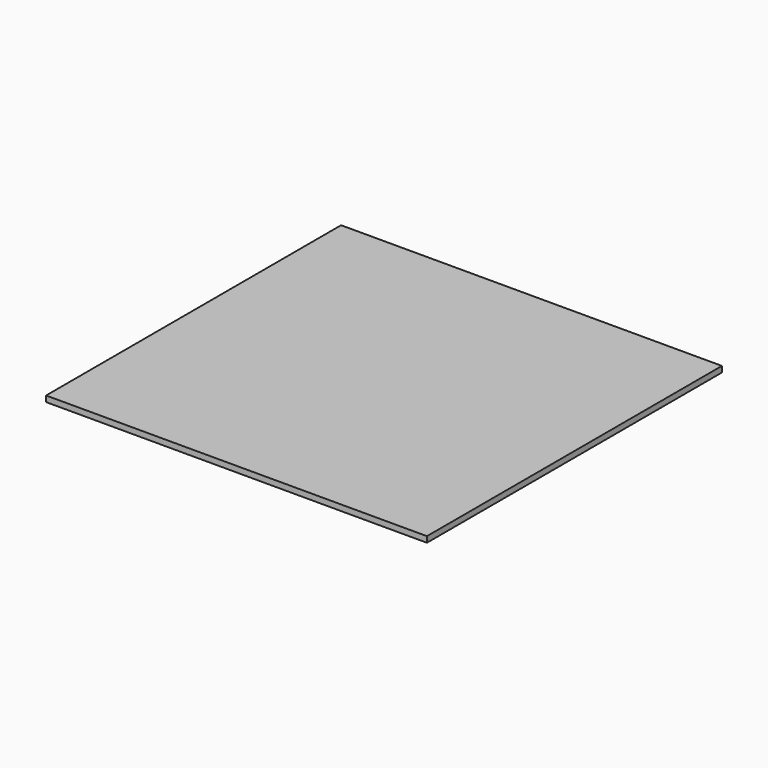
from build123d import *

# Parameters (mm, degrees)
F0_W     = 207.14430511
F0_H     = 200.555562973
F1_DEPTH = 3.175


# Not quite as in the source:
# - a length typed as a fraction of an inch, garbled in the dataset ("3 / 203.2 mm" for 3/8 in), is restored


with BuildPart() as f1:
    # F0 (on Top) → F1 (new body)
    with BuildSketch(Plane.XY):
        Rectangle(F0_W, F0_H)
    extrude(amount=F1_DEPTH)


solid = f1.part
